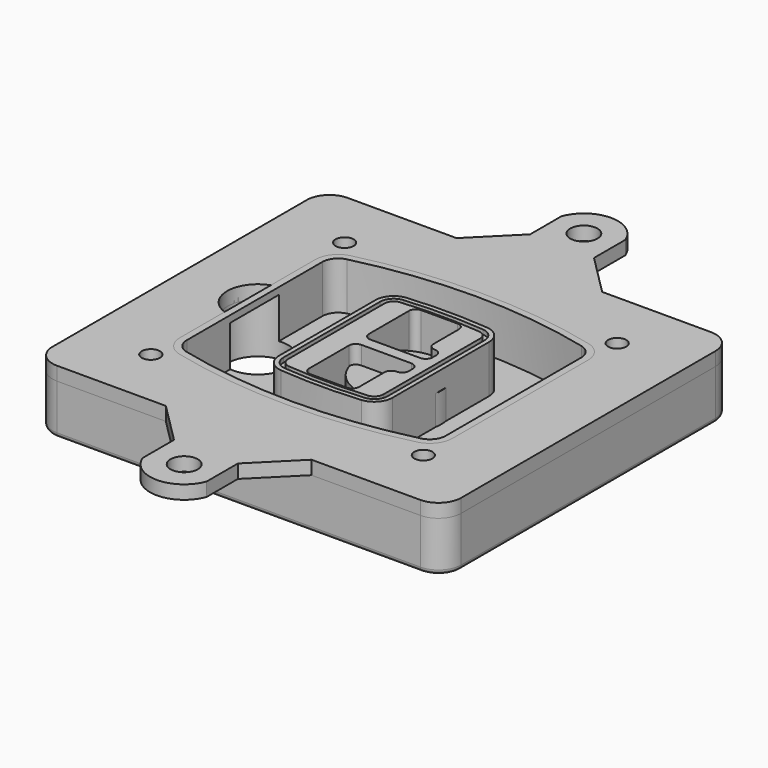
from build123d import *

# Parameters (mm, degrees)
F0_R      = 4
F1_DEPTH  = 25
F2_DEPTH  = 3
F3_DEPTH  = 18
F5_DEPTH  = 21
F6_DEPTH  = 2
F8_DEPTH  = 20
F9_DEPTH  = 16
F10_DEPTH = 25
F7_R      = 6
F7_R_2    = 4
F11_DEPTH = 6
F13_DEPTH = 9
F15_R     = 2
F16_R     = 6
F16_R_2   = 4
F17_DEPTH = 3


# Not quite as in the source:
# - a feature of the source that left no trace in its solid (it failed there, or was rolled back) is left out
# - a feature names something its author has since deleted; it is built from what else it names


with BuildPart() as f1:
    # F0 (on Top) → F1 (new body)
    with BuildSketch(Plane.XY):
        with BuildLine():
            ThreePointArc((-90, -70), (-87.0710678119, -77.0710678119), (-80, -80))
            Line((-80, -80), (80, -80))
            ThreePointArc((80, -80), (87.0710678119, -77.0710678119), (90, -70))
            Line((90, -70), (90, 70))
            ThreePointArc((90, 70), (87.0710678119, 77.0710678119), (80, 80))
            Line((80, 80), (-80, 80))
            ThreePointArc((-80, 80), (-87.0710678119, 77.0710678119), (-90, 70))
            Line((-90, 70), (-90, -70))
        make_face()
        with Locations((-60, -53.3333333333)):
            Circle(F0_R, mode=Mode.SUBTRACT)
        with Locations((60, -53.3333333333)):
            Circle(F0_R, mode=Mode.SUBTRACT)
        with Locations((-60, 53.3333333333)):
            Circle(F0_R, mode=Mode.SUBTRACT)
        with BuildLine():
            ThreePointArc((-64, 37.2990447398), (-61.0143011354, 45.9411029726), (-53.3306899286, 50.8970778549))
            ThreePointArc((-53.3306899286, 50.8970778549), (0, 57.3333333333), (53.3306899286, 50.8970778549))
            ThreePointArc((53.3306899286, 50.8970778549), (61.0143011354, 45.9411029726), (64, 37.2990447398))
            Line((64, 37.2990447398), (64, -37.2990447398))
            ThreePointArc((64, -37.2990447398), (61.0143011354, -45.9411029726), (53.3306899286, -50.8970778549))
            ThreePointArc((53.3306899286, -50.8970778549), (0, -57.3333333333), (-53.3306899286, -50.8970778549))
            ThreePointArc((-53.3306899286, -50.8970778549), (-61.0143011354, -45.9411029726), (-64, -37.2990447398))
            Line((-64, -37.2990447398), (-64, 37.2990447398))
        make_face(mode=Mode.SUBTRACT)
        with Locations((60, 53.3333333333)):
            Circle(F0_R, mode=Mode.SUBTRACT)
        with BuildLine():
            ThreePointArc((53.3306899286, 50.8970778549), (0, 57.3333333333), (-53.3306899286, 50.8970778549))
            ThreePointArc((-53.3306899286, 50.8970778549), (-61.0143011354, 45.9411029726), (-64, 37.2990447398))
            Line((-64, 37.2990447398), (-64, -37.2990447398))
            ThreePointArc((-64, -37.2990447398), (-61.0143011354, -45.9411029726), (-53.3306899286, -50.8970778549))
            ThreePointArc((-53.3306899286, -50.8970778549), (0, -57.3333333333), (53.3306899286, -50.8970778549))
            ThreePointArc((53.3306899286, -50.8970778549), (61.0143011354, -45.9411029726), (64, -37.2990447398))
            Line((64, -37.2990447398), (64, 37.2990447398))
            ThreePointArc((64, 37.2990447398), (61.0143011354, 45.9411029726), (53.3306899286, 50.8970778549))
        make_face()
        with BuildLine():
            Line((-60, -37.2990447398), (-60, 37.2990447398))
            ThreePointArc((-60, 37.2990447398), (-57.8673579538, 43.4719434775), (-52.3790642347, 47.0119255363))
            ThreePointArc((-52.3790642347, 47.0119255363), (0, 53.3333333333), (52.3790642347, 47.0119255363))
            ThreePointArc((52.3790642347, 47.0119255363), (57.8673579538, 43.4719434775), (60, 37.2990447398))
            Line((60, 37.2990447398), (60, -37.2990447398))
            ThreePointArc((60, -37.2990447398), (57.8673579538, -43.4719434775), (52.3790642347, -47.0119255363))
            ThreePointArc((52.3790642347, -47.0119255363), (0, -53.3333333333), (-52.3790642347, -47.0119255363))
            ThreePointArc((-52.3790642347, -47.0119255363), (-57.8673579538, -43.4719434775), (-60, -37.2990447398))
        make_face(mode=Mode.SUBTRACT)
        with BuildLine():
            ThreePointArc((-52.3790642347, 47.0119255363), (-57.8673579538, 43.4719434775), (-60, 37.2990447398))
            Line((-60, 37.2990447398), (-60, -37.2990447398))
            ThreePointArc((-60, -37.2990447398), (-57.8673579538, -43.4719434775), (-52.3790642347, -47.0119255363))
            ThreePointArc((-52.3790642347, -47.0119255363), (0, -53.3333333333), (52.3790642347, -47.0119255363))
            ThreePointArc((52.3790642347, -47.0119255363), (57.8673579538, -43.4719434775), (60, -37.2990447398))
            Line((60, -37.2990447398), (60, 37.2990447398))
            ThreePointArc((60, 37.2990447398), (57.8673579538, 43.4719434775), (52.3790642347, 47.0119255363))
            ThreePointArc((52.3790642347, 47.0119255363), (0, 53.3333333333), (-52.3790642347, 47.0119255363))
        make_face()
        with BuildLine():
            ThreePointArc((51.6653449643, 44.0980612973), (55.5071505677, 41.6200738562), (57, 37.2990447398))
            Line((57, 37.2990447398), (57, -37.2990447398))
            ThreePointArc((57, -37.2990447398), (55.5071505677, -41.6200738562), (51.6653449643, -44.0980612973))
            ThreePointArc((51.6653449643, -44.0980612973), (0, -50.3333333333), (-51.6653449643, -44.0980612973))
            ThreePointArc((-51.6653449643, -44.0980612973), (-55.5071505677, -41.6200738562), (-57, -37.2990447398))
            Line((-57, -37.2990447398), (-57, 37.2990447398))
            ThreePointArc((-57, 37.2990447398), (-55.5071505677, 41.6200738562), (-51.6653449643, 44.0980612973))
            ThreePointArc((-51.6653449643, 44.0980612973), (0, 50.3333333333), (51.6653449643, 44.0980612973))
        make_face(mode=Mode.SUBTRACT)
        with BuildLine():
            Line((57, -37.2990447398), (57, 37.2990447398))
            ThreePointArc((57, 37.2990447398), (55.5071505677, 41.6200738562), (51.6653449643, 44.0980612973))
            ThreePointArc((51.6653449643, 44.0980612973), (0, 50.3333333333), (-51.6653449643, 44.0980612973))
            ThreePointArc((-51.6653449643, 44.0980612973), (-55.5071505677, 41.6200738562), (-57, 37.2990447398))
            Line((-57, 37.2990447398), (-57, -37.2990447398))
            ThreePointArc((-57, -37.2990447398), (-55.5071505677, -41.6200738562), (-51.6653449643, -44.0980612973))
            ThreePointArc((-51.6653449643, -44.0980612973), (0, -50.3333333333), (51.6653449643, -44.0980612973))
            ThreePointArc((51.6653449643, -44.0980612973), (55.5071505677, -41.6200738562), (57, -37.2990447398))
        make_face()
    extrude(amount=-F1_DEPTH)

    # F0 (on Top) → F2 (join)
    with BuildSketch(Plane.XY):
        with BuildLine():
            ThreePointArc((-52.3790642347, 47.0119255363), (-57.8673579538, 43.4719434775), (-60, 37.2990447398))
            Line((-60, 37.2990447398), (-60, -37.2990447398))
            ThreePointArc((-60, -37.2990447398), (-57.8673579538, -43.4719434775), (-52.3790642347, -47.0119255363))
            ThreePointArc((-52.3790642347, -47.0119255363), (0, -53.3333333333), (52.3790642347, -47.0119255363))
            ThreePointArc((52.3790642347, -47.0119255363), (57.8673579538, -43.4719434775), (60, -37.2990447398))
            Line((60, -37.2990447398), (60, 37.2990447398))
            ThreePointArc((60, 37.2990447398), (57.8673579538, 43.4719434775), (52.3790642347, 47.0119255363))
            ThreePointArc((52.3790642347, 47.0119255363), (0, 53.3333333333), (-52.3790642347, 47.0119255363))
        make_face()
        with BuildLine():
            ThreePointArc((51.6653449643, 44.0980612973), (55.5071505677, 41.6200738562), (57, 37.2990447398))
            Line((57, 37.2990447398), (57, -37.2990447398))
            ThreePointArc((57, -37.2990447398), (55.5071505677, -41.6200738562), (51.6653449643, -44.0980612973))
            ThreePointArc((51.6653449643, -44.0980612973), (0, -50.3333333333), (-51.6653449643, -44.0980612973))
            ThreePointArc((-51.6653449643, -44.0980612973), (-55.5071505677, -41.6200738562), (-57, -37.2990447398))
            Line((-57, -37.2990447398), (-57, 37.2990447398))
            ThreePointArc((-57, 37.2990447398), (-55.5071505677, 41.6200738562), (-51.6653449643, 44.0980612973))
            ThreePointArc((-51.6653449643, 44.0980612973), (0, 50.3333333333), (51.6653449643, 44.0980612973))
        make_face(mode=Mode.SUBTRACT)
    extrude(amount=F2_DEPTH)

    # F0 (on Top) → F3 (cut)
    with BuildSketch(Plane.XY):
        with BuildLine():
            Line((57, -37.2990447398), (57, 37.2990447398))
            ThreePointArc((57, 37.2990447398), (55.5071505677, 41.6200738562), (51.6653449643, 44.0980612973))
            ThreePointArc((51.6653449643, 44.0980612973), (0, 50.3333333333), (-51.6653449643, 44.0980612973))
            ThreePointArc((-51.6653449643, 44.0980612973), (-55.5071505677, 41.6200738562), (-57, 37.2990447398))
            Line((-57, 37.2990447398), (-57, -37.2990447398))
            ThreePointArc((-57, -37.2990447398), (-55.5071505677, -41.6200738562), (-51.6653449643, -44.0980612973))
            ThreePointArc((-51.6653449643, -44.0980612973), (0, -50.3333333333), (51.6653449643, -44.0980612973))
            ThreePointArc((51.6653449643, -44.0980612973), (55.5071505677, -41.6200738562), (57, -37.2990447398))
        make_face()
    extrude(amount=-F3_DEPTH, mode=Mode.SUBTRACT)

    # F4 (on face) → F5 (join, through all)
    with BuildSketch(Plane.XY.offset(3)):
        with BuildLine():
            ThreePointArc((-25, -26.587695628), (-22.8992979869, -31.9912392117), (-17.7004291845, -34.5569740744))
            ThreePointArc((-17.7004291845, -34.5569740744), (0, -35.3333333333), (17.7004291845, -34.5569740744))
            ThreePointArc((17.7004291845, -34.5569740744), (22.8992979869, -31.9912392117), (25, -26.587695628))
            Line((25, -26.587695628), (25, 26.587695628))
            ThreePointArc((25, 26.587695628), (22.8992979869, 31.9912392117), (17.7004291845, 34.5569740744))
            ThreePointArc((17.7004291845, 34.5569740744), (0, 35.3333333333), (-17.7004291845, 34.5569740744))
            ThreePointArc((-17.7004291845, 34.5569740744), (-22.8992979869, 31.9912392117), (-25, 26.587695628))
            Line((-25, 26.587695628), (-25, -26.587695628))
        make_face()
        with BuildLine():
            ThreePointArc((17.5253218884, 32.5646544628), (21.4244734902, 30.6403533158), (23, 26.587695628))
            Line((23, 26.587695628), (23, -26.587695628))
            ThreePointArc((23, -26.587695628), (21.4244734902, -30.6403533158), (17.5253218884, -32.5646544628))
            ThreePointArc((17.5253218884, -32.5646544628), (0, -33.3333333333), (-17.5253218884, -32.5646544628))
            ThreePointArc((-17.5253218884, -32.5646544628), (-21.4244734902, -30.6403533158), (-23, -26.587695628))
            Line((-23, -26.587695628), (-23, 26.587695628))
            ThreePointArc((-23, 26.587695628), (-21.4244734902, 30.6403533158), (-17.5253218884, 32.5646544628))
            ThreePointArc((-17.5253218884, 32.5646544628), (0, 33.3333333333), (17.5253218884, 32.5646544628))
        make_face(mode=Mode.SUBTRACT)
        with BuildLine():
            Line((23, -26.587695628), (23, 26.587695628))
            ThreePointArc((23, 26.587695628), (21.4244734902, 30.6403533158), (17.5253218884, 32.5646544628))
            ThreePointArc((17.5253218884, 32.5646544628), (0, 33.3333333333), (-17.5253218884, 32.5646544628))
            ThreePointArc((-17.5253218884, 32.5646544628), (-21.4244734902, 30.6403533158), (-23, 26.587695628))
            Line((-23, 26.587695628), (-23, -26.587695628))
            ThreePointArc((-23, -26.587695628), (-21.4244734902, -30.6403533158), (-17.5253218884, -32.5646544628))
            ThreePointArc((-17.5253218884, -32.5646544628), (0, -33.3333333333), (17.5253218884, -32.5646544628))
            ThreePointArc((17.5253218884, -32.5646544628), (21.4244734902, -30.6403533158), (23, -26.587695628))
        make_face()
        with BuildLine():
            ThreePointArc((17.3502145923, 30.5723348512), (19.9496489934, 29.2894674198), (21, 26.587695628))
            Line((21, 26.587695628), (21, -26.587695628))
            ThreePointArc((21, -26.587695628), (19.9496489934, -29.2894674198), (17.3502145923, -30.5723348512))
            ThreePointArc((17.3502145923, -30.5723348512), (0, -31.3333333333), (-17.3502145923, -30.5723348512))
            ThreePointArc((-17.3502145923, -30.5723348512), (-19.9496489934, -29.2894674198), (-21, -26.587695628))
            Line((-21, -26.587695628), (-21, 26.587695628))
            ThreePointArc((-21, 26.587695628), (-19.9496489934, 29.2894674198), (-17.3502145923, 30.5723348512))
            ThreePointArc((-17.3502145923, 30.5723348512), (0, 31.3333333333), (17.3502145923, 30.5723348512))
        make_face(mode=Mode.SUBTRACT)
        with BuildLine():
            Line((21, -26.587695628), (21, 26.587695628))
            ThreePointArc((21, 26.587695628), (19.9496489934, 29.2894674198), (17.3502145923, 30.5723348512))
            ThreePointArc((17.3502145923, 30.5723348512), (0, 31.3333333333), (-17.3502145923, 30.5723348512))
            ThreePointArc((-17.3502145923, 30.5723348512), (-19.9496489934, 29.2894674198), (-21, 26.587695628))
            Line((-21, 26.587695628), (-21, -26.587695628))
            ThreePointArc((-21, -26.587695628), (-19.9496489934, -29.2894674198), (-17.3502145923, -30.5723348512))
            ThreePointArc((-17.3502145923, -30.5723348512), (0, -31.3333333333), (17.3502145923, -30.5723348512))
            ThreePointArc((17.3502145923, -30.5723348512), (19.9496489934, -29.2894674198), (21, -26.587695628))
        make_face()
        with BuildLine():
            Line((-8, -2.5), (14, -2.5))
            ThreePointArc((14, -2.5), (16.1213203436, -3.3786796564), (17, -5.5))
            Line((17, -5.5), (17, -7.5))
            ThreePointArc((17, -7.5), (16.1213203436, -9.6213203436), (14, -10.5))
            ThreePointArc((14, -10.5), (11.8786796564, -11.3786796564), (11, -13.5))
            Line((11, -13.5), (11, -27.5))
            ThreePointArc((11, -27.5), (10.1213203436, -29.6213203436), (8, -30.5))
            Line((8, -30.5), (-8, -30.5))
            ThreePointArc((-8, -30.5), (-10.1213203436, -29.6213203436), (-11, -27.5))
            Line((-11, -27.5), (-11, -5.5))
            ThreePointArc((-11, -5.5), (-10.1213203436, -3.3786796564), (-8, -2.5))
        make_face(mode=Mode.SUBTRACT)
        with BuildLine():
            ThreePointArc((-8, 2.5), (-10.1213203436, 3.3786796564), (-11, 5.5))
            Line((-11, 5.5), (-11, 27.5))
            ThreePointArc((-11, 27.5), (-10.1213203436, 29.6213203436), (-8, 30.5))
            Line((-8, 30.5), (8, 30.5))
            ThreePointArc((8, 30.5), (10.1213203436, 29.6213203436), (11, 27.5))
            Line((11, 27.5), (11, 13.5))
            ThreePointArc((11, 13.5), (11.8786796564, 11.3786796564), (14, 10.5))
            ThreePointArc((14, 10.5), (16.1213203436, 9.6213203436), (17, 7.5))
            Line((17, 7.5), (17, 5.5))
            ThreePointArc((17, 5.5), (16.1213203436, 3.3786796564), (14, 2.5))
            Line((14, 2.5), (-8, 2.5))
        make_face(mode=Mode.SUBTRACT)
    extrude(amount=-F5_DEPTH)

    # F4 (on face) → F6 (cut)
    with BuildSketch(Plane.XY.offset(3)):
        with BuildLine():
            Line((23, -26.587695628), (23, 26.587695628))
            ThreePointArc((23, 26.587695628), (21.4244734902, 30.6403533158), (17.5253218884, 32.5646544628))
            ThreePointArc((17.5253218884, 32.5646544628), (0, 33.3333333333), (-17.5253218884, 32.5646544628))
            ThreePointArc((-17.5253218884, 32.5646544628), (-21.4244734902, 30.6403533158), (-23, 26.587695628))
            Line((-23, 26.587695628), (-23, -26.587695628))
            ThreePointArc((-23, -26.587695628), (-21.4244734902, -30.6403533158), (-17.5253218884, -32.5646544628))
            ThreePointArc((-17.5253218884, -32.5646544628), (0, -33.3333333333), (17.5253218884, -32.5646544628))
            ThreePointArc((17.5253218884, -32.5646544628), (21.4244734902, -30.6403533158), (23, -26.587695628))
        make_face()
        with BuildLine():
            ThreePointArc((17.3502145923, 30.5723348512), (19.9496489934, 29.2894674198), (21, 26.587695628))
            Line((21, 26.587695628), (21, -26.587695628))
            ThreePointArc((21, -26.587695628), (19.9496489934, -29.2894674198), (17.3502145923, -30.5723348512))
            ThreePointArc((17.3502145923, -30.5723348512), (0, -31.3333333333), (-17.3502145923, -30.5723348512))
            ThreePointArc((-17.3502145923, -30.5723348512), (-19.9496489934, -29.2894674198), (-21, -26.587695628))
            Line((-21, -26.587695628), (-21, 26.587695628))
            ThreePointArc((-21, 26.587695628), (-19.9496489934, 29.2894674198), (-17.3502145923, 30.5723348512))
            ThreePointArc((-17.3502145923, 30.5723348512), (0, 31.3333333333), (17.3502145923, 30.5723348512))
        make_face(mode=Mode.SUBTRACT)
    extrude(amount=-F6_DEPTH, mode=Mode.SUBTRACT)

    # F7 (on face) → F8 (join)
    with BuildSketch(Plane(origin=(0, 0, -25), x_dir=(1, 0, 0), z_dir=(0, 0, -1))):
        with BuildLine():
            ThreePointArc((-6.71157564, 0), (6.7567035675, 13.4682792075), (20.224982775, 0))
            Line((20.224982775, 0), (25.224982775, 0))
            ThreePointArc((25.224982775, 0), (6.7567035675, 18.4682792075), (-11.71157564, 0))
            Line((-11.71157564, 0), (-6.71157564, 0))
        make_face()
        with BuildLine():
            Line((-6.71157564, 0), (20.224982775, 0))
            ThreePointArc((20.224982775, 0), (6.7567035675, 13.4682792075), (-6.71157564, 0))
        make_face()
        with BuildLine():
            ThreePointArc((-6.71157564, 0), (6.7567035675, -13.4682792075), (20.224982775, 0))
            Line((20.224982775, 0), (-6.71157564, 0))
        make_face()
        with BuildLine():
            Line((25.224982775, 0), (20.224982775, 0))
            ThreePointArc((20.224982775, 0), (6.7567035675, -13.4682792075), (-6.71157564, 0))
            Line((-6.71157564, 0), (-11.71157564, 0))
            ThreePointArc((-11.71157564, 0), (6.7567035675, -18.4682792075), (25.224982775, 0))
        make_face()
    extrude(amount=-F8_DEPTH)

    # F7 (on face) → F9 (cut)
    with BuildSketch(Plane(origin=(0, 0, -25), x_dir=(1, 0, 0), z_dir=(0, 0, -1))):
        with BuildLine():
            Line((-6.71157564, 0), (20.224982775, 0))
            ThreePointArc((20.224982775, 0), (6.7567035675, 13.4682792075), (-6.71157564, 0))
        make_face()
        with BuildLine():
            ThreePointArc((-6.71157564, 0), (6.7567035675, -13.4682792075), (20.224982775, 0))
            Line((20.224982775, 0), (-6.71157564, 0))
        make_face()
    extrude(amount=-F9_DEPTH, mode=Mode.SUBTRACT)

    # F7 (on face) → F10 (cut)
    with BuildSketch(Plane(origin=(0, 0, -25), x_dir=(1, 0, 0), z_dir=(0, 0, -1))):
        with BuildLine():
            Line((-69.0318229325, 0), (-42.0952645175, 0))
            ThreePointArc((-42.0952645175, 0), (-55.563543725, 13.4682792075), (-69.0318229325, 0))
        make_face()
        with BuildLine():
            ThreePointArc((-69.0318229325, 0), (-55.563543725, -13.4682792075), (-42.0952645175, 0))
            Line((-42.0952645175, 0), (-69.0318229325, 0))
        make_face()
    extrude(amount=-F10_DEPTH, mode=Mode.SUBTRACT)

    # F7 (on face) → F11 (cut)
    with BuildSketch(Plane(origin=(0, 0, -25), x_dir=(1, 0, 0), z_dir=(0, 0, -1))):
        with Locations((60, -53.3333333333)):
            Circle(F7_R)
        with Locations((60, -53.3333333333)):
            Circle(F7_R_2, mode=Mode.SUBTRACT)
        with Locations((-60, -53.3333333333)):
            Circle(F7_R)
        with Locations((-60, -53.3333333333)):
            Circle(F7_R_2, mode=Mode.SUBTRACT)
        with Locations((-60, 53.3333333333)):
            Circle(F7_R)
        with Locations((-60, 53.3333333333)):
            Circle(F7_R_2, mode=Mode.SUBTRACT)
        with Locations((60, 53.3333333333)):
            Circle(F7_R)
        with Locations((60, 53.3333333333)):
            Circle(F7_R_2, mode=Mode.SUBTRACT)
    extrude(amount=-F11_DEPTH, mode=Mode.SUBTRACT)

    # F12 (on face) → F13 (cut, through all)
    with BuildSketch(Plane(origin=(0, 0, -9), x_dir=(1, 0, 0), z_dir=(0, 0, -1))):
        with BuildLine():
            ThreePointArc((20.224982775, 0), (20.1663399806, 1.2554664788), (19.9909222755, 2.5))
            Line((19.9909222755, 2.5), (14, 2.5))
            ThreePointArc((14, 2.5), (16.1213203436, 3.3786796564), (17, 5.5))
            Line((17, 5.5), (17, 7.5))
            ThreePointArc((17, 7.5), (16.1213203436, 9.6213203436), (14, 10.5))
            ThreePointArc((14, 10.5), (12.1627255951, 11.1284134507), (11.0951631559, 12.750384826))
            ThreePointArc((11.0951631559, 12.750384826), (11.0476113807, 12.7664660322), (11, 12.7823698976))
            Line((11, 12.7823698976), (11, -12.7823698976))
            ThreePointArc((11, -12.7823698976), (11.0476113807, -12.7664660322), (11.0951631559, -12.750384826))
            ThreePointArc((11.0951631559, -12.750384826), (12.1627255951, -11.1284134507), (14, -10.5))
            ThreePointArc((14, -10.5), (16.1213203436, -9.6213203436), (17, -7.5))
            Line((17, -7.5), (17, -5.5))
            ThreePointArc((17, -5.5), (16.1213203436, -3.3786796564), (14, -2.5))
            Line((14, -2.5), (19.9909222755, -2.5))
            ThreePointArc((19.9909222755, -2.5), (20.1663399806, -1.2554664788), (20.224982775, 0))
        make_face()
    extrude(amount=F13_DEPTH, mode=Mode.SUBTRACT)

    # F15
    f15_edges = [f1.edges().sort_by_distance(p)[0] for p in [
        (0, -80, -25),
        (-87.071068, -77.071068, -25),
        (-90, 0, -25),
        (-87.071068, 77.071068, -25),
        (87.071068, -77.071068, -25),
        (0, 80, -25),
        (90, 0, -25),
        (87.071068, 77.071068, -25),
    ]]
    fillet(f15_edges, radius=F15_R)


with BuildPart() as f17:
    # F16 (on face) → F17 (new body, symmetric)
    with BuildSketch(Plane.XY):
        with BuildLine():
            ThreePointArc((14.0598719019, 115.2268539391), (0, 125), (-14.0598719019, 115.2268539391))
            Line((-14.0598719019, 115.2268539391), (-14.0598719019, 98))
            Line((-14.0598719019, 98), (-32.0598719019, 80))
            Line((-32.0598719019, 80), (32.0598719019, 80))
            Line((32.0598719019, 80), (14.0598719019, 98))
            Line((14.0598719019, 98), (14.0598719019, 115.2268539391))
        make_face()
        with Locations((0, 110)):
            Circle(F16_R, mode=Mode.SUBTRACT)
        with BuildLine():
            Line((32.0598719019, 80), (-32.0598719019, 80))
            Line((-32.0598719019, 80), (-80, 80))
            ThreePointArc((-80, 80), (-87.0710678119, 77.0710678119), (-90, 70))
            Line((-90, 70), (-90, -70))
            ThreePointArc((-90, -70), (-87.0710678119, -77.0710678119), (-80, -80))
            Line((-80, -80), (-32.0598719019, -80))
            Line((-32.0598719019, -80), (32.0598719019, -80))
            Line((32.0598719019, -80), (80, -80))
            ThreePointArc((80, -80), (87.0710678119, -77.0710678119), (90, -70))
            Line((90, -70), (90, 70))
            ThreePointArc((90, 70), (87.0710678119, 77.0710678119), (80, 80))
            Line((80, 80), (32.0598719019, 80))
        make_face()
        with Locations((-60, -53.3333333333)):
            Circle(F16_R_2, mode=Mode.SUBTRACT)
        with BuildLine():
            ThreePointArc((-60, 37.2990447398), (-57.8673579538, 43.4719434775), (-52.3790642347, 47.0119255363))
            ThreePointArc((-52.3790642347, 47.0119255363), (0, 53.3333333333), (52.3790642347, 47.0119255363))
            ThreePointArc((52.3790642347, 47.0119255363), (57.8673579538, 43.4719434775), (60, 37.2990447398))
            Line((60, 37.2990447398), (60, -37.2990447398))
            ThreePointArc((60, -37.2990447398), (57.8673579538, -43.4719434775), (52.3790642347, -47.0119255363))
            ThreePointArc((52.3790642347, -47.0119255363), (0, -53.3333333333), (-52.3790642347, -47.0119255363))
            ThreePointArc((-52.3790642347, -47.0119255363), (-57.8673579538, -43.4719434775), (-60, -37.2990447398))
            Line((-60, -37.2990447398), (-60, -12.7166190685))
            ThreePointArc((-60, -12.7166190685), (-66.5441169481, -7.798817635), (-69.0318229325, 0))
            ThreePointArc((-69.0318229325, 0), (-66.5441169481, 7.798817635), (-60, 12.7166190685))
            Line((-60, 12.7166190685), (-60, 37.2990447398))
        make_face(mode=Mode.SUBTRACT)
        with Locations((60, -53.3333333333)):
            Circle(F16_R_2, mode=Mode.SUBTRACT)
        with Locations((-60, 53.3333333333)):
            Circle(F16_R_2, mode=Mode.SUBTRACT)
        with Locations((60, 53.3333333333)):
            Circle(F16_R_2, mode=Mode.SUBTRACT)
        with BuildLine():
            Line((32.0598719019, -80), (-32.0598719019, -80))
            Line((-32.0598719019, -80), (-14.0598719019, -98))
            Line((-14.0598719019, -98), (-14.0598719019, -115.2268539391))
            ThreePointArc((-14.0598719019, -115.2268539391), (0, -125), (14.0598719019, -115.2268539391))
            Line((14.0598719019, -115.2268539391), (14.0598719019, -98))
            Line((14.0598719019, -98), (32.0598719019, -80))
        make_face()
        with Locations((0, -110)):
            Circle(F16_R, mode=Mode.SUBTRACT)
    extrude(amount=F17_DEPTH, both=True)


solid = Compound([f1.part, f17.part])
